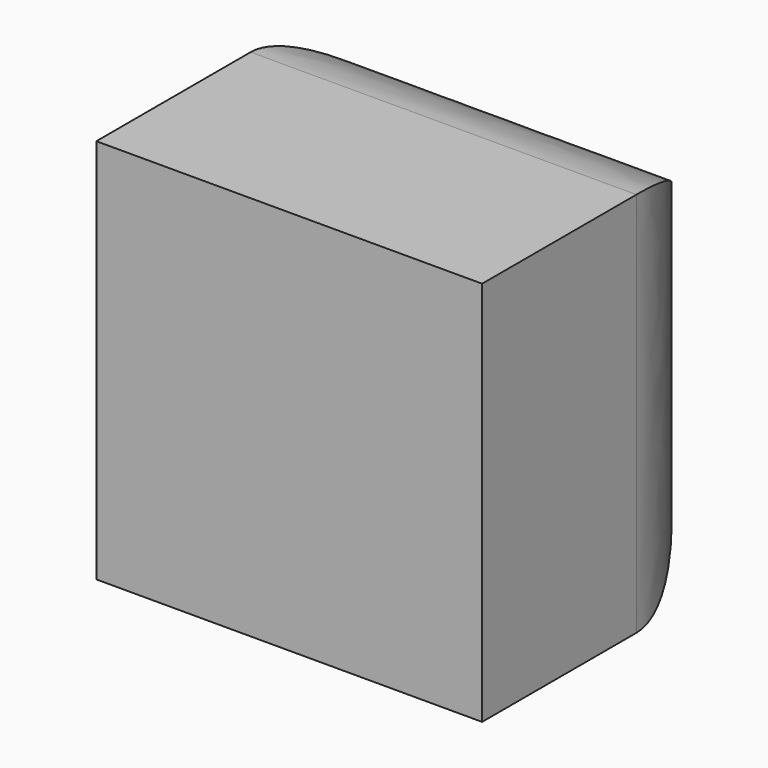
from build123d import *

# Parameters (mm, degrees)
F0_W        = 12.7
F0_H        = 25.4
F1_DEPTH    = 25.4
F2_T1_DEPTH = 88.9
F2_T3_DEPTH = 88.9


# Not quite as in the source:
# - a fillet or chamfer that OpenCascade refuses, or shapes differently, is made with other operations: its cross-section is extruded or revolved along the edge and cut away or added


with BuildPart() as f1:
    # F0 (on Top) → F1 (new body)
    with BuildSketch(Plane.XY):
        with Locations((-6.35, 12.7)):
            Rectangle(F0_W, F0_H)
        with Locations((6.35, 12.7)):
            Rectangle(F0_W, F0_H)
    extrude(amount=F1_DEPTH)

    # F2: fillet of radius 12.7 on 4 edges, made by hand

    # F2_s2 → F2_t1 (cut)
    with BuildSketch(Plane.XY.offset(-31.75)):
        with BuildLine():
            add(Edge.make_bspline(
                [(12.7, 12.7), (12.7, 25.4), (0, 25.4)],
                knots=[0, 0, 0, 1, 1, 1], degree=2, weights=[1, 0.4285714286, 1]))
            Line((0, 25.4), (12.7, 25.4))
            Line((12.7, 25.4), (12.7, 12.7))
        make_face()
        with BuildLine():
            add(Edge.make_bspline(
                [(-12.7, 12.7), (-12.7, 25.4), (0, 25.4)],
                knots=[0, 0, 0, 1, 1, 1], degree=2, weights=[1, 0.4285714286, 1]))
            Line((0, 25.4), (-12.7, 25.4))
            Line((-12.7, 25.4), (-12.7, 12.7))
        make_face()
    extrude(amount=F2_T1_DEPTH, mode=Mode.SUBTRACT)

    # F2_s4 → F2_t3 (cut)
    with BuildSketch(Plane.YZ.offset(-44.45)):
        with BuildLine():
            add(Edge.make_bspline(
                [(25.4, 12.7), (25.4, 0), (12.7, 0)],
                knots=[0, 0, 0, 1, 1, 1], degree=2, weights=[1, 0.4285714286, 1]))
            Line((12.7, 0), (25.4, 0))
            Line((25.4, 0), (25.4, 12.7))
        make_face()
        with BuildLine():
            add(Edge.make_bspline(
                [(25.4, 12.7), (25.4, 25.4), (12.7, 25.4)],
                knots=[0, 0, 0, 1, 1, 1], degree=2, weights=[1, 0.4285714286, 1]))
            Line((12.7, 25.4), (25.4, 25.4))
            Line((25.4, 25.4), (25.4, 12.7))
        make_face()
    extrude(amount=F2_T3_DEPTH, mode=Mode.SUBTRACT)


solid = f1.part
